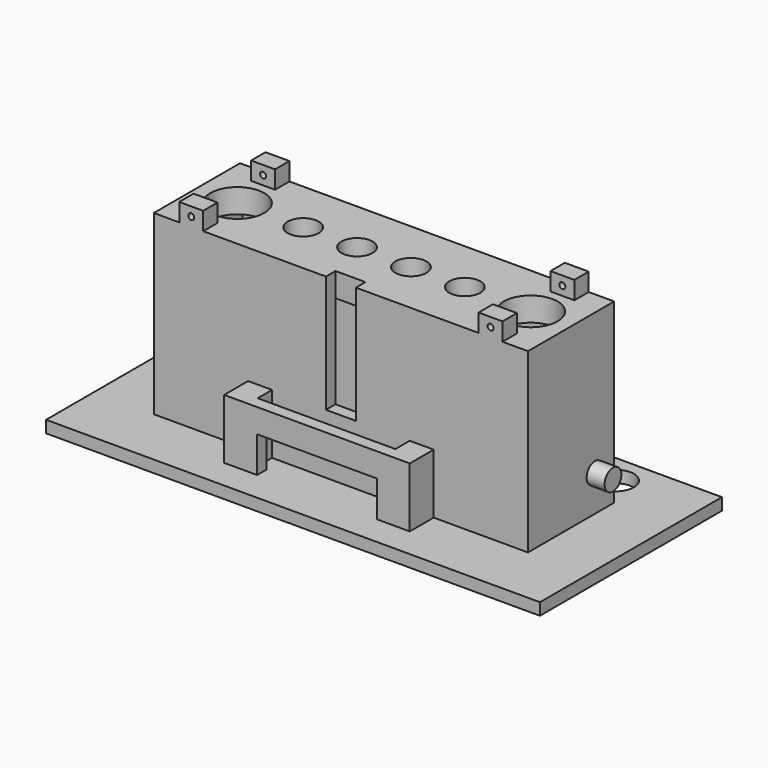
from build123d import *

# Parameters (mm, degrees)
F1_DEPTH  = 31.6
F2_START  = 27.6
F2_DEPTH  = 4
F0_R      = 3.05
F3_DEPTH  = 2
F4_W      = 2.5
F4_H      = 19.6
F5_DEPTH  = 2
F7_DEPTH  = 3
F8_R      = 0.5
F9_DEPTH  = 25
F10_R     = 1.75
F11_DEPTH = 3
F13_DEPTH = 10
F15_DEPTH = 4


# Not quite as in the source:
# - a feature names something its author has since deleted; it is built from what else it names


with BuildPart() as f1:
    # F0 (on Top) → F1 (new body)
    with BuildSketch(Plane.XY):
        Polygon((31.25, -9), (31.25, 0), (29.25, 0), (29.25, -7), (-29.25, -7), (-29.25, 0), (-31.25, 0), (-31.25, -9), align=None)
        Polygon((31.25, 0), (31.25, 9), (-31.25, 9), (-31.25, 0), (-29.25, 0), (-29.25, 7), (29.25, 7), (29.25, 0), align=None)
    extrude(amount=F1_DEPTH)

    # F0 (on Top) → F2 (join)
    with BuildSketch(Plane.XY.offset(F2_START)):
        with BuildLine():
            Line((29, 0), (29.25, 0))
            Line((29.25, 0), (29.25, 7))
            Line((29.25, 7), (-29.25, 7))
            Line((-29.25, 7), (-29.25, 0))
            Line((-29.25, 0), (-29, 0))
            ThreePointArc((-29, 0), (-24.5, 4.5), (-20, 0))
            Line((-20, 0), (-16.1, 0))
            ThreePointArc((-16.1, 0), (-13.5, 2.6), (-10.9, 0))
            Line((-10.9, 0), (-7.1, 0))
            ThreePointArc((-7.1, 0), (-4.5, 2.6), (-1.9, 0))
            Line((-1.9, 0), (0, 0))
            Line((0, 0), (1.9, 0))
            ThreePointArc((1.9, 0), (4.5, 2.6), (7.1, 0))
            Line((7.1, 0), (10.9, 0))
            ThreePointArc((10.9, 0), (13.5, 2.6), (16.1, 0))
            Line((16.1, 0), (20, 0))
            ThreePointArc((20, 0), (24.5, 4.5), (29, 0))
        make_face()
        with BuildLine():
            Line((29.25, -7), (29.25, 0))
            Line((29.25, 0), (29, 0))
            ThreePointArc((29, 0), (24.5, -4.5), (20, 0))
            Line((20, 0), (16.1, 0))
            ThreePointArc((16.1, 0), (13.5, -2.6), (10.9, 0))
            Line((10.9, 0), (7.1, 0))
            ThreePointArc((7.1, 0), (4.5, -2.6), (1.9, 0))
            Line((1.9, 0), (0, 0))
            Line((0, 0), (-1.9, 0))
            ThreePointArc((-1.9, 0), (-4.5, -2.6), (-7.1, 0))
            Line((-7.1, 0), (-10.9, 0))
            ThreePointArc((-10.9, 0), (-13.5, -2.6), (-16.1, 0))
            Line((-16.1, 0), (-20, 0))
            ThreePointArc((-20, 0), (-24.5, -4.5), (-29, 0))
            Line((-29, 0), (-29.25, 0))
            Line((-29.25, 0), (-29.25, -7))
            Line((-29.25, -7), (29.25, -7))
        make_face()
    extrude(amount=F2_DEPTH)

    # F0 (on Top) → F3 (join)
    with BuildSketch(Plane.XY):
        Polygon((-41.25, 19), (-41.25, 14), (-41.25, -19), (41.25, -19), (41.25, 19), align=None)
        with Locations((-27.5, 14)):
            Circle(F0_R, mode=Mode.SUBTRACT)
        Polygon((-31.25, 9), (31.25, 9), (31.25, 0), (31.25, -9), (-31.25, -9), (-31.25, 0), align=None, mode=Mode.SUBTRACT)
        with Locations((27.5, 14)):
            Circle(F0_R, mode=Mode.SUBTRACT)
    extrude(amount=F3_DEPTH)

    # F4 (on face) → F5 (cut)
    with BuildSketch(Plane.XZ.offset(9)):
        with Locations((-1.25, 21.8)):
            Rectangle(F4_W, F4_H)
        with Locations((1.25, 21.8)):
            Rectangle(F4_W, F4_H)
    extrude(amount=-F5_DEPTH, mode=Mode.SUBTRACT)

    # F6 (on face) → F7 (join)
    with BuildSketch(Plane.XY.offset(31.6)):
        Polygon((-27, -6), (-27, -9), (-25, -9), (-23, -9), (-23, -6), (-25, -6), align=None)
        Polygon((23, -6), (23, -9), (25, -9), (27, -9), (27, -6), (25, -6), align=None)
        Polygon((-23, 6), (-23, 9), (-25, 9), (-27, 9), (-27, 6), (-25, 6), align=None)
        Polygon((25, 6), (27, 6), (27, 9), (25, 9), (23, 9), (23, 6), align=None)
    extrude(amount=F7_DEPTH)

    # F8 (on face) → F9 (cut)
    with BuildSketch(Plane.XZ.offset(9)):
        with BuildLine():
            ThreePointArc((-25, 33.6), (-25.3535533906, 32.7464466094), (-24.5, 33.1))
            ThreePointArc((-24.5, 33.1), (-24.6464466094, 33.4535533906), (-25, 33.6))
        make_face()
        with Locations((25, 33.1)):
            Circle(F8_R)
    extrude(amount=-F9_DEPTH, mode=Mode.SUBTRACT)

    # F10 (on face) → F11 (join)
    with BuildSketch(Plane.YZ.offset(31.25)):
        with Locations((5, 8)):
            Circle(F10_R)
    extrude(amount=F11_DEPTH)

    # F12 (on face) → F13 (join)
    with BuildSketch(Plane.XY.offset(2)):
        Polygon((-11.5, -9), (-15.5, -9), (-15.5, -11), (-15.5, -14), (0, -14), (15.5, -14), (15.5, -11), (15.5, -9), (11.5, -9), (11.5, -12), (0, -12), (-11.5, -12), align=None)
    extrude(amount=F13_DEPTH)

    # F14 (on face) → F15 (cut)
    with BuildSketch(Plane.XZ.offset(14)):
        Polygon((-10, 2), (0, 2), (10, 2), (10, 8), (0, 8), (-10, 8), align=None)
    extrude(amount=-F15_DEPTH, mode=Mode.SUBTRACT)


solid = f1.part
